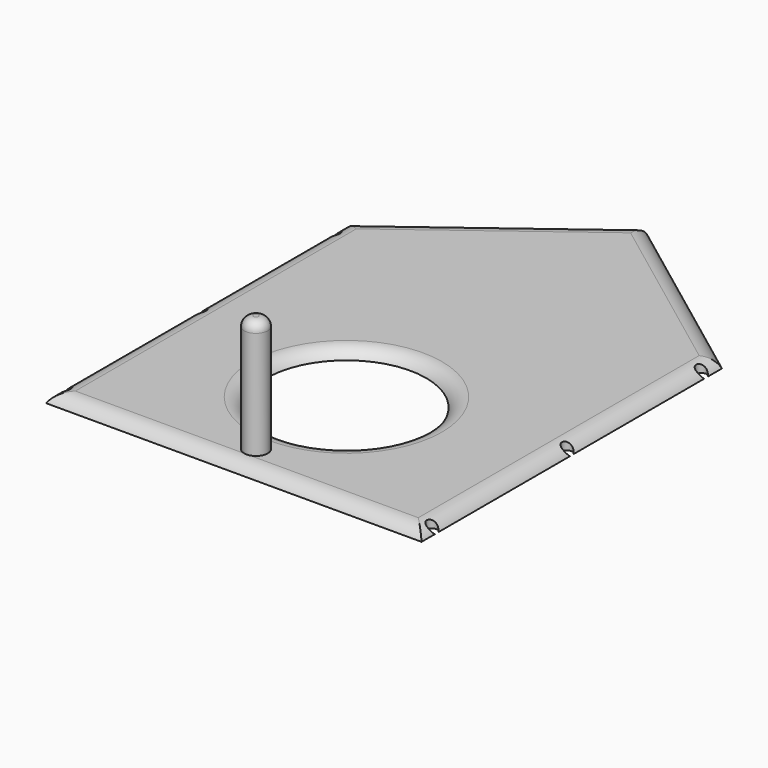
from build123d import *

# Parameters (mm, degrees)
F0_W         = 101.6
F0_H         = 101.6
F0_R         = 21.59
F1_DEPTH     = 2.54
F3_R         = 3.175
F4_DEPTH     = 31.75
F5_R         = 2.54
F6_T1_DEPTH  = 123.5970452561
F6_T3_DEPTH  = 85.4970452561
F6_T5_DEPTH  = 85.4970452561
F6_T10_DEPTH = 123.5970452561
F6_S11_R     = 3.175
F6_T12_DEPTH = 63
F8_D         = 2.794


# Not quite as in the source:
# - a fillet or chamfer that OpenCascade refuses, or shapes differently, is made with other operations: its cross-section is extruded or revolved along the edge and cut away or added


with BuildPart() as f1:
    # F0 (on Top) → F1 (new body)
    with BuildSketch(Plane.XY):
        Rectangle(F0_W, F0_H)
        with Locations((0, -12.7)):
            Circle(F0_R, mode=Mode.SUBTRACT)
        Polygon((-50.8, 50.8), (50.8, 50.8), (0, 88.9), align=None)
    extrude(amount=F1_DEPTH)

    # F2: fillet of radius 4.826 on 1 edges, made by hand

    # F2_s1 → F2_t2 (revolve, cut)
    with BuildSketch(Plane.XZ.offset(12.7)):
        with BuildLine():
            ThreePointArc((21.59, 0), (23.3645471712, 1.8566146333), (25.8402329348, 2.54))
            Line((25.8402329348, 2.54), (21.59, 2.54))
            Line((21.59, 2.54), (21.59, 0))
        make_face()
    revolve(axis=Axis((0, -12.7, 2.54), (0, 0, 1)), mode=Mode.SUBTRACT)

    # F3 (on face) → F4 (join)
    with BuildSketch(Plane.XY.offset(2.54)):
        with Locations((0, -43.2976202148)):
            Circle(F3_R)
    extrude(amount=F4_DEPTH)

    # F5
    f5_edges = [f1.edges().sort_by_distance(p)[0] for p in [
        (-3.175, -43.29762, 34.29),
    ]]
    fillet(f5_edges, radius=F5_R)

    # F6: fillet of radius 5.08 on 5 edges, made by hand

    # F6_s2 → F6_t1 (cut)
    with BuildSketch(Plane.XZ.offset(-61.7985226281)):
        with BuildLine():
            ThreePointArc((46.4005909488, 2.54), (48.9405909488, 1.8594090512), (50.8, 0))
            Line((50.8, 0), (50.8, 2.54))
            Line((50.8, 2.54), (46.4005909488, 2.54))
        make_face()
        with BuildLine():
            ThreePointArc((-46.4005909488, 2.54), (-48.9405909488, 1.8594090512), (-50.8, 0))
            Line((-50.8, 0), (-50.8, 2.54))
            Line((-50.8, 2.54), (-46.4005909488, 2.54))
        make_face()
    extrude(amount=F6_T1_DEPTH, mode=Mode.SUBTRACT)

    # F6_s4 → F6_t3 (cut)
    with BuildSketch(Plane(origin=(51.4708181025, 38.6031135768, 0), x_dir=(0, 0, 1), z_dir=(-0.8, -0.6, 0))):
        with BuildLine():
            ThreePointArc((2.54, 66.7205909488), (1.8594090512, 69.2605909488), (0, 71.12))
            Line((0, 71.12), (2.54, 71.12))
            Line((2.54, 71.12), (2.54, 66.7205909488))
        make_face()
    extrude(amount=F6_T3_DEPTH, mode=Mode.SUBTRACT)

    # F6_s6 → F6_t5 (cut)
    with BuildSketch(Plane(origin=(16.9268181025, -12.6951135768, 0), x_dir=(0, 0, 1), z_dir=(-0.8, 0.6, 0))):
        with BuildLine():
            ThreePointArc((2.54, 66.7205909488), (1.8594090512, 69.2605909488), (0, 71.12))
            Line((0, 71.12), (2.54, 71.12))
            Line((2.54, 71.12), (2.54, 66.7205909488))
        make_face()
    extrude(amount=F6_T5_DEPTH, mode=Mode.SUBTRACT)


with BuildPart() as f6_tool8:
    # F6_s9 → F6_t10 (new body)
    with BuildSketch(Plane.YZ.offset(-61.7985226281)):
        with BuildLine():
            ThreePointArc((-46.4005909488, 2.54), (-48.9405909488, 1.8594090512), (-50.8, 0))
            Line((-50.8, 0), (-50.8, 2.54))
            Line((-50.8, 2.54), (-46.4005909488, 2.54))
        make_face()
    extrude(amount=F6_T10_DEPTH)

    # F6_s11 → F6_t12 (cut, symmetric)
    with BuildSketch(Plane.XY.offset(1.3)):
        with Locations((0, -43.2976202148)):
            Circle(F6_S11_R)
    extrude(amount=F6_T12_DEPTH, both=True, mode=Mode.SUBTRACT)


with BuildPart() as f1_1:
    add(f1.part)

    # F6_t7: cut F6_tool8
    add(f6_tool8.part, mode=Mode.SUBTRACT)

    # F8 (through all)
    with Locations(Plane(origin=(0, 0, 0), x_dir=(1, 0, 0), z_dir=(0, 0, -1))):
        with Locations((-49.53, -45.4025), (-49.53, 0), (-49.53, 45.72), (49.53, 45.72), (49.53, 0), (49.53, -45.4025)):
            Hole(F8_D / 2)


solid = f1_1.part
